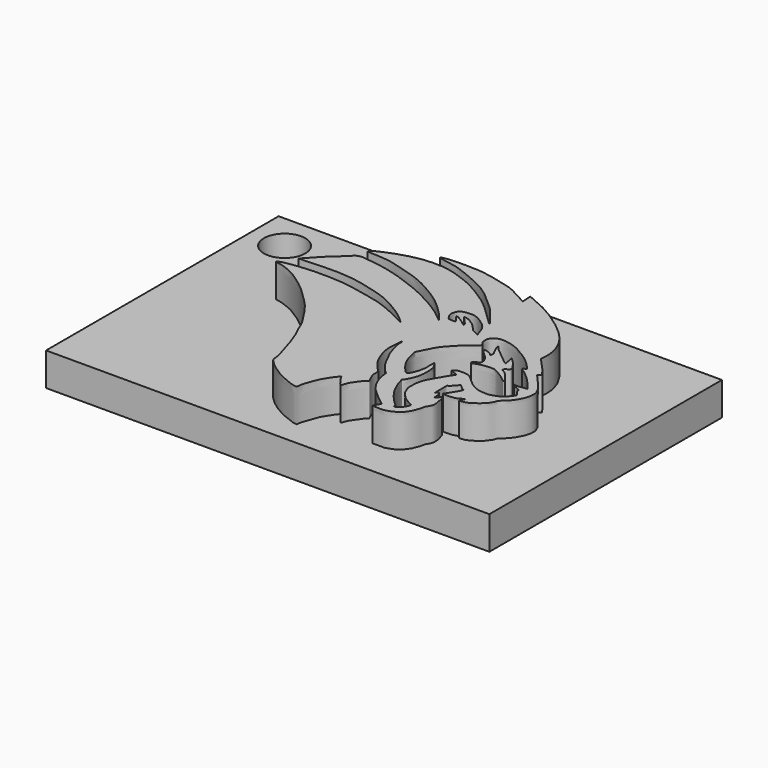
from build123d import *

# Parameters (mm, degrees)
F1_DEPTH = 25.4
F2_W     = 169.9344962835
F2_H     = 111.438959837
F3_DEPTH = 12.7
F4_R     = 7.9340721322
F5_DEPTH = 12.7


with BuildPart() as f1:
    # F0 (on Top) → F1 (new body)
    with BuildSketch(Plane.XY):
        with BuildLine():
            add(Edge.make_bspline(
                [(-14.8701705039, -19.9608001858), (-15.221690835, -19.2073334084), (-16.625382793, -16.9660551756), (-18.8145764823, -13.5974487599), (-21.7376055558, -9.4480503555), (-24.5386587115, -6.7651875872), (-29.2213836952, -2.0490323537), (-33.2090632506, 1.0266070698), (-37.3108516979, 3.8703194609), (-40.8750632464, 5.4725585398), (-43.1505063811, 6.3712258286), (-45.6984791671, 6.6961246185), (-46.2951241921, 7.0290269329), (-44.8273788111, 7.882301282), (-39.360546355, 8.6917755145), (-34.1503227711, 9.2199630692), (-26.1459287774, 9.1377803946), (-20.0552998643, 8.7078848215), (-11.5265680921, 6.7838277487), (-3.8234144736, 5.439385618), (7.2025946105, -0.1900501111), (7.7620278934, -0.5655499869), (4.9446039361, 2.0869717823), (1.3008896446, 4.7134534316), (-6.2511301784, 9.1315364238), (-13.4707319379, 10.9498852738), (-20.6605380633, 12.8767111483), (-30.7241335125, 13.5705283972), (-42.4874100153, 12.5018346524), (-41.7984071827, 12.9505929764), (-37.5569983073, 18.1037160515), (-31.7015431097, 22.7550582109), (-29.4633653878, 25.8033399973), (-24.708812529, 25.0026945191), (-20.5160586827, 24.5677127931), (-15.2447575815, 23.3952223693), (-11.1346154852, 22.1707374066), (-6.0005872173, 20.2473769611), (-1.6724236886, 18.5603562875), (2.331046156, 16.6096027421), (8.29978858, 13.3578117406), (12.9239596286, 10.140973274), (15.6933934459, 7.6938469217), (15.6850383581, 7.89041196), (13.883384297, 10.090120142), (12.2058740691, 12.0633831707), (8.2658950795, 15.7571136876), (5.1340905457, 18.2144922263), (0.5632813688, 21.0207749349), (-6.4295798331, 25.0167682013), (-16.519293927, 27.6010671806), (-19.6579640118, 28.5861202918), (-23.8244520748, 28.9321353102), (-27.5500194279, 29.1854619589), (-29.16994936, 29.0672202828), (-28.1023726327, 30.353145993), (-24.7800008778, 32.0217797709), (-18.8741048653, 34.1780204807), (-13.5989570646, 35.3844069692), (-9.0323236761, 35.7835224645), (-2.9568390979, 35.6441536417), (3.3871239944, 33.4430463754), (8.2582535453, 31.6254999822), (14.6988445903, 27.7308645526), (19.9782008784, 24.093188458), (24.8414343333, 19.1570210972), (29.0842273756, 15.1532805254), (29.0583545521, 15.3743411164), (27.8326579227, 17.2644078083), (25.9216038578, 19.4174660639), (23.0912459993, 23.2704910801), (19.4803048629, 26.0157171151), (16.9172953139, 28.7464960896), (12.009652843, 32.3100804683), (7.8786740384, 34.205264408), (-0.2201321112, 37.689521901), (-3.738465721, 38.5113119793), (-9.5098774215, 39.3772960778), (-9.2770451577, 39.8608323233), (-6.9503719579, 40.6697590859), (2.1658518543, 40.6240338322), (8.3670057819, 40.2357657644), (15.9816872911, 38.1517431998), (20.0146961816, 37.4251070757), (27.8026964381, 32.7643186249), (27.6739209409, 32.9274427311), (27.3919925021, 36.7329457257), (27.5484843103, 36.8192611002), (32.4487131354, 34.6740896565), (36.6415975911, 32.7362745493), (42.7969610095, 28.7852221639), (48.5775150448, 24.268635265), (52.9337999958, 19.280053861), (55.0956073548, 13.8730755246), (55.4842683059, 10.1023036419), (55.0875139263, 7.1366526371), (55.3311692316, 7.1202657281), (57.7038333216, 4.5151308529), (60.3403166523, 1.7873756635), (61.939783591, -0.7081872431), (61.9228089872, -0.8086404409), (60.574069747, -1.7619053144), (61.0873702539, -1.7516944394), (63.4024083186, -4.654014828), (66.17166014, -7.5165247573), (68.1323436188, -10.9753429081), (67.8403103062, -13.1464579427), (67.6210421965, -15.0307386106), (65.640256939, -18.8574840013), (63.7104902718, -20.7455148396), (61.9313019034, -22.131081262), (62.1416817304, -22.4638249746), (60.8967608126, -25.0173278873), (58.6701119256, -26.9078061444), (55.6505064167, -29.1445212539), (52.9064282632, -29.200166737), (52.8306873093, -28.9601536167), (54.2587664847, -26.6717106228), (53.8839650384, -27.2313234607), (51.986947732, -28.202550438), (50.6863481156, -28.8914707136), (46.3013264955, -28.9387192384), (46.5333158111, -28.5869206357), (50.3248376243, -22.7564692567), (49.2210127604, -22.7158735399), (48.185540697, -22.0953245327), (47.1820811341, -20.9209510008), (47.0179091111, -20.9423835074), (46.6610780555, -21.5222448894), (45.2715282704, -23.1642257164), (44.167485725, -23.8633478866), (44.0402199406, -24.056182696), (44.1077165563, -29.7391059746), (44.2424677108, -29.704882972), (44.9298643008, -28.6712101943), (44.9381784477, -28.8370782507), (45.5831789496, -29.401201917), (45.864978196, -30.2230405033), (45.8332800239, -32.2718499355), (46.0431048441, -32.2755521981), (47.4692449016, -30.6316210775), (47.5469474527, -30.6892542641), (48.1762281967, -31.282144751), (48.371150022, -32.9354354483), (49.2512481663, -36.4603778502), (47.3811785445, -38.5688666877), (47.4524172153, -39.4615142051), (46.5083937337, -42.4569406109), (44.8959673155, -45.3657836507), (41.914363728, -47.2577489049), (39.0930786202, -48.2934718337), (34.795474344, -47.9571483407), (34.6768461287, -47.8599376798), (36.1959801627, -45.3084678781), (36.1902562655, -45.2579861076), (33.7606289335, -43.4890994336), (31.005504084, -41.0736791631), (29.0903946087, -39.4485380637), (27.0544984579, -36.7124973539), (26.2052841843, -34.8407220549), (25.3516880158, -32.9031814643), (24.8613111568, -30.2531084511), (24.8021921451, -28.8153721599), (24.6122776651, -28.8230825397), (23.104162879, -27.4433091425), (21.7153959083, -25.6768723498), (20.4329502947, -23.8892225341), (18.6964093559, -20.1452708334), (17.2594231542, -17.5956807998), (16.6237447114, -14.5308822773), (15.7251002718, -12.5388593615), (15.9159556833, -9.7175450977), (15.5207961884, -9.7228985059), (15.3609709913, -13.0420997075), (15.0656157152, -16.1703142138), (16.0186872903, -20.1187864391), (17.4136983079, -23.5588760784), (18.9549102776, -25.9436355229), (21.9758647632, -29.3687856007), (22.3569011856, -29.4518910165), (22.2376625902, -31.1794785211), (22.4750841628, -33.0583982423), (24.0202604041, -35.8112373772), (23.9463212602, -36.028333464), (22.5757336735, -36.9887746178), (20.943115437, -39.6377331191), (19.7932835549, -40.972712028), (19.3189891957, -43.2705295118), (19.0892741552, -43.458963868), (18.4627295862, -43.0816932453), (17.8686520769, -42.1261702125), (17.0528733375, -41.1679156433), (16.109135116, -39.7611917977), (15.6583942757, -38.8552512589), (15.6104844294, -38.9871019848), (14.3312472417, -40.4613756955), (13.3504238678, -41.9874928854), (11.8584359055, -44.2493834769), (11.0665219392, -46.3231070406), (10.3429374422, -48.4545552842), (9.5481856978, -50.5759957274), (9.4060648235, -52.6403351753), (9.2664064233, -52.548184411), (7.3118521794, -52.2554939359), (6.1305638917, -51.7591076991), (4.0715548368, -50.9332182637), (2.6639768562, -50.3066956696), (0.3932070477, -49.2283306871), (-0.8310979, -48.3336778562), (-2.7127827276, -47.1310762319), (-4.0555159667, -46.1714522576), (-5.3632720538, -45.0356818132), (-6.4975041884, -43.8850295891), (-7.182897798, -43.1226518866), (-7.380134713, -41.7532388731), (-7.4756957962, -39.8994589754), (-8.5070257448, -36.9732060036), (-9.2147602073, -34.1386657639), (-10.8225901787, -29.4048978612), (-12.0411906467, -26.0805747104), (-14.3615500092, -21.5481532407), (-14.6179117826, -20.5015045177), (-14.8701705039, -19.9608001858)],
                knots=[0, 0, 0, 0, 0.0049590764, 0.0106061426, 0.016680571, 0.0221570205, 0.0291463365, 0.035406483, 0.041507596, 0.0468596575, 0.0512669827, 0.0555951815, 0.0572286385, 0.0601650163, 0.0665969859, 0.0731046834, 0.0807298933, 0.0876144071, 0.0954411961, 0.1038200224, 0.1131017527, 0.1140904599, 0.118810238, 0.1250375053, 0.1330476617, 0.1405539476, 0.1478284981, 0.1572094569, 0.1658855329, 0.1669309593, 0.1738224901, 0.1816783163, 0.1866466719, 0.1922969184, 0.1980883273, 0.2043697068, 0.2101110067, 0.2164930184, 0.2223771807, 0.2281425874, 0.2352554764, 0.2421856215, 0.2468671041, 0.2473346344, 0.2516558946, 0.2564592041, 0.2627017487, 0.2682262867, 0.2744074888, 0.282384837, 0.2911494078, 0.2961304728, 0.3016781712, 0.3071340679, 0.3098696002, 0.3125796856, 0.3179116131, 0.324879731, 0.3312527163, 0.3370665617, 0.3437997703, 0.3508469281, 0.3571476255, 0.3645737848, 0.3715184541, 0.3791939238, 0.3852229214, 0.385690448, 0.3895207526, 0.3944300134, 0.4003918346, 0.4061884017, 0.4115376563, 0.4181101703, 0.4242049613, 0.4321048907, 0.4379816572, 0.4440887567, 0.4451444794, 0.4490539196, 0.4573399172, 0.4645212824, 0.4718608605, 0.4782035884, 0.485915255, 0.4863827815, 0.4917402097, 0.4925264925, 0.4984560343, 0.5048101093, 0.5121024041, 0.5195938822, 0.5266301668, 0.5331279162, 0.538695168, 0.543034523, 0.5439975213, 0.5488290373, 0.5547449555, 0.5590731578, 0.5599045546, 0.5631786289, 0.5642240637, 0.5692763645, 0.5751173705, 0.5804194282, 0.5842950202, 0.5880583314, 0.5936498687, 0.5984342584, 0.602204778, 0.6035864923, 0.607914847, 0.6128095051, 0.6182308748, 0.6223969879, 0.6234527164, 0.6276280473, 0.6287400235, 0.6326366055, 0.636509555, 0.6418817611, 0.6430348398, 0.6500227568, 0.651870568, 0.6550343659, 0.658344166, 0.659153963, 0.6612392578, 0.6654028881, 0.6683692991, 0.6700051711, 0.676433051, 0.6769005775, 0.6798574986, 0.6804134934, 0.6827741764, 0.6856180495, 0.6893619372, 0.6901717169, 0.6941813883, 0.6948425707, 0.6971056628, 0.700695022, 0.7058660708, 0.7101646546, 0.7126665176, 0.7173844792, 0.7224741508, 0.7274362617, 0.7325236684, 0.7379167078, 0.7386158231, 0.7432876129, 0.7439487953, 0.7483990214, 0.7538993845, 0.7582783917, 0.7632614867, 0.7671915517, 0.7711550361, 0.775803219, 0.7788079417, 0.7796956946, 0.7834272361, 0.7876800285, 0.7917488674, 0.7972703082, 0.8020637783, 0.8067614762, 0.8110937967, 0.8153825704, 0.8161923588, 0.8208585152, 0.8260444454, 0.8314992394, 0.8366829416, 0.8416135651, 0.8472610284, 0.8487320422, 0.8520050943, 0.8561718649, 0.8608311889, 0.8618869239, 0.8652254355, 0.8701156049, 0.8739784356, 0.8779832805, 0.8791663401, 0.881313675, 0.8842410479, 0.8873494754, 0.89107548, 0.8935398956, 0.8940958815, 0.8977306082, 0.9016935172, 0.9061340889, 0.9102387251, 0.9142950107, 0.9186718845, 0.9222837622, 0.9229449498, 0.9266313029, 0.9300288983, 0.9339769443, 0.9375023646, 0.9417549496, 0.9452196622, 0.949250475, 0.9528113421, 0.9564191576, 0.9598913133, 0.9626013979, 0.9657002356, 0.9694549995, 0.974203598, 0.9789962015, 0.9850087791, 0.9904260981, 0.9964412577, 1, 1, 1, 1], degree=3))
        make_face()
        with BuildLine():
            add(Edge.make_bspline(
                [(29.4968672097, -24.9577090144), (29.2522813062, -24.9043141851), (28.4812583162, -24.3288345548), (27.5929491341, -23.2719328433), (26.5229917254, -21.9955450296), (25.493437854, -20.5251037399), (24.6801994651, -18.8995632069), (23.7965645353, -16.7549151809), (23.5446819954, -15.2740390303), (22.8719216364, -12.7119711385), (23.1418972942, -12.5584518565), (24.0154471471, -10.7766411032), (24.8407424624, -9.0693079132), (25.7289367901, -7.3485281619), (26.6559375418, -5.7613972679), (27.9062254963, -4.402126541), (29.3948903999, -2.6292634603), (31.343901089, -0.7824786076), (33.0107668247, 0.5689504112), (36.0390233406, 3.1686364904), (35.9834240148, 3.2841340245), (35.6347872021, 3.8315916102), (35.005968941, 4.300492855), (34.7946306934, 4.9794904566), (34.5639802183, 5.7982686669), (34.6727768135, 7.0835200419), (34.8494314161, 7.7637528325), (35.94184202, 8.8377452141), (36.7700559773, 9.3848304088), (38.0363565573, 9.6500972977), (39.3511875283, 9.7145928207), (40.869122491, 9.4131606486), (42.3186128653, 9.1230203463), (44.026639396, 8.5857606938), (45.8727467194, 7.68829074), (47.8396434221, 6.5647391811), (49.8921781905, 5.215646461), (51.5848538888, 4.0321336566), (52.9695426633, 2.8273251949), (53.9756652747, 1.9079844198), (54.8974443301, 0.9258478712), (56.0933963356, -0.5431734266), (56.0207767113, -0.5670851704), (54.1235992374, -1.2246906294), (56.2822414189, -2.2455961102), (57.6365652943, -3.4384410011), (59.3846260322, -4.8281482901), (61.5253326842, -7.1508611227), (62.8766661704, -8.6414132572), (64.2432189508, -10.4720364135), (64.1997307341, -10.526147049), (59.7430846208, -11.0959072724), (59.7174238209, -10.9952495415), (59.6902079837, -11.4932703081), (59.9344673636, -11.454688787), (60.6232913696, -11.7775056805), (61.9410395375, -12.3229908584), (62.6393846502, -12.5961227275), (62.6889607213, -12.6094395811), (62.6625293454, -13.4198997169), (62.9036332557, -13.6998131955), (63.4146030144, -14.6248848381), (64.2644012778, -15.4843576067), (64.2703472473, -15.7514541503), (63.9234444764, -16.361517992), (63.4297453755, -17.0077291171), (62.7483134067, -17.9428439939), (61.9461286613, -18.6920912439), (60.8047053901, -19.4764804344), (59.610563815, -19.9893153206), (58.3977560095, -20.3972567855), (57.1621739162, -20.7127926969), (54.2515411403, -20.5373729033), (52.545532541, -20.0953776823), (51.4815664159, -19.5692402803), (49.810596204, -18.671860239), (48.4987708398, -17.5074042444), (47.2886545958, -16.4657526062), (45.9680404199, -15.1378893551), (44.7528113291, -14.4934294299), (44.0590602712, -14.2394496595), (41.5424638767, -14.1212587014), (40.1505333119, -14.2608331208), (38.9793963625, -15.4409237635), (39.1237154987, -15.4063690401), (41.8773489728, -16.5324190222), (41.8239116772, -16.6685628078), (40.7814556828, -18.1805789408), (39.8307999292, -19.7584860445), (38.1065802723, -22.8115033724), (36.8276457119, -24.8247273526), (36.0353024844, -27.1936372084), (35.8496389089, -29.0603054241), (35.7335787494, -32.1031719848), (36.2453574344, -33.2884937889), (36.8904467346, -35.167947655), (38.2553679411, -36.6942464133), (39.4521075695, -37.8586499835), (41.1618511172, -39.1545600075), (42.6344482129, -39.8792255326), (43.5349553427, -40.2601234265), (43.6672085696, -40.3228808223), (43.3143919959, -41.291093515), (42.7961663324, -42.4471597398), (41.9537717412, -43.4601082839), (39.9286333798, -44.6437510012), (39.9618076609, -44.5526966368), (40.2143745036, -43.8364478953), (40.3769174243, -43.7835236104), (39.7876396563, -43.1654184035), (38.7768422844, -42.3758353972), (37.5647722531, -41.1135438714), (35.985791676, -39.4389294723), (34.8617251798, -37.7398674458), (33.7240328862, -36.1555212265), (32.5232966552, -33.6359437906), (31.7177003126, -31.7152639125), (31.0803960041, -29.2030854921), (31.027858707, -29.0871536111), (31.9380822088, -28.4634787891), (32.6092110474, -26.791776108), (33.3562917023, -25.1762993701), (33.6960741144, -23.6231477851), (33.9665612048, -21.6674261934), (33.8939165999, -19.4673360972), (33.7027397946, -17.7752237335), (33.3178878557, -16.5192743382), (31.8672968177, -14.4640934143), (31.9505985192, -14.7443602135), (31.8170442568, -16.2400374977), (31.9924971318, -18.777125191), (31.7811989512, -19.7408665822), (31.528565593, -21.2958227698), (31.1066790709, -22.4766680866), (30.6997434225, -23.6613789894), (29.9457354274, -24.859026972), (29.6448590614, -24.9900166803), (29.4968672097, -24.9577090144)],
                knots=[0, 0, 0, 0, 0.006708734, 0.0144130343, 0.0226490646, 0.0311626116, 0.039890883, 0.0493826184, 0.057895195, 0.0677654799, 0.0709231679, 0.0795607269, 0.0887905781, 0.097612174, 0.1062196534, 0.11485172, 0.1246327534, 0.1348342225, 0.1452057541, 0.1573642731, 0.1589999693, 0.1639254641, 0.1697072445, 0.1749195449, 0.1808782163, 0.1880129868, 0.193429241, 0.2011293672, 0.2076153379, 0.2147148113, 0.2220925584, 0.2299864519, 0.237772496, 0.2462695547, 0.2554227104, 0.2650908387, 0.2751205536, 0.2843744603, 0.2929782354, 0.3002602254, 0.3082835034, 0.3165615666, 0.317684609, 0.3249480775, 0.3327687674, 0.3418661817, 0.351408113, 0.3626123005, 0.3725114042, 0.3814704885, 0.3825935316, 0.3961282686, 0.397072702, 0.4010824118, 0.4036885486, 0.4091333639, 0.417180781, 0.4223604778, 0.4234835209, 0.4289134912, 0.4330069073, 0.4396236854, 0.4465657437, 0.4495595445, 0.4546913699, 0.4606197317, 0.4674303071, 0.4741699253, 0.4816466722, 0.488986991, 0.4960523262, 0.5033082496, 0.514206795, 0.5227193748, 0.5295815911, 0.5383182275, 0.5468204757, 0.5549256413, 0.5637399519, 0.5710041943, 0.5765496675, 0.5864616594, 0.5946376019, 0.6020108916, 0.6034230767, 0.6143949758, 0.6162049256, 0.6243221211, 0.6336315891, 0.6454446706, 0.6555491241, 0.6653333321, 0.67437203, 0.6852890022, 0.6926242463, 0.7014522327, 0.7105702363, 0.7188843537, 0.7282076754, 0.7366805764, 0.742645227, 0.7444812104, 0.7505381602, 0.7578489963, 0.7658296409, 0.775006834, 0.7758982315, 0.7814648168, 0.783617228, 0.7888689744, 0.7963361757, 0.8048163339, 0.8145443315, 0.8236276266, 0.8325853264, 0.8430582674, 0.8530497307, 0.8628253522, 0.8646080832, 0.8706988281, 0.8795016982, 0.8880478532, 0.8960344579, 0.905024029, 0.9145835946, 0.9226851084, 0.9307244732, 0.9400188431, 0.9415627396, 0.9492835742, 0.9596791693, 0.9661358264, 0.9739811762, 0.9811886388, 0.9884938738, 0.9959407392, 1, 1, 1, 1], degree=3))
        make_face(mode=Mode.SUBTRACT)
        with BuildLine():
            add(Edge.make_bspline(
                [(20.6397492439, 14.123653993), (20.9231291787, 14.107879862), (21.8316466788, 13.93482722), (23.1814379486, 13.2319928397), (24.2685977622, 12.5031395213), (25.2851042185, 11.8029468382), (26.4551056622, 10.4876070808), (27.0116800828, 9.9606050571), (27.651520023, 9.0647820094), (27.6538790026, 9.0845364936), (30.3610957538, 7.7412480397), (30.524767696, 7.7040205885), (30.4572964756, 8.0451735726), (30.1223764768, 9.0581679563), (29.5146238145, 10.7117994099), (28.9519533833, 12.0465400778), (27.7826519006, 13.3927760879), (26.8076966332, 14.1959491787), (25.5528714349, 15.1491849512), (24.249629435, 15.8970217765), (22.9819249355, 16.5507416428), (21.4841487521, 16.9479582393), (19.0832462787, 16.799759965), (17.8153748373, 16.5130973878), (16.8876470254, 15.9476291337), (16.3799579835, 15.2221343774), (16.0716009629, 14.4413838238), (15.8556372224, 12.9644797308), (16.2875433013, 11.8733345043), (16.6705653081, 11.1557862317), (17.4821370215, 10.366983682), (17.3319115827, 10.0971338051), (20.2859489837, 10.0363455976), (20.185530873, 10.1749470183), (19.9675570561, 10.5040692491), (19.4825241559, 11.3400304848), (18.935412513, 11.8704385213), (18.4480258577, 12.6144128586), (18.1808939016, 13.0607831433), (18.1662521839, 13.1213895313), (18.9230205816, 13.0032916053), (20.5270821027, 12.0237739131), (21.4184918676, 11.3544149547), (23.3070051117, 9.9365483519), (23.4059621734, 10.0067156562), (23.570445725, 10.4381450188), (22.713484547, 11.3464290964), (21.8490601971, 12.439939261), (21.0915870868, 13.162654499), (20.4832637271, 13.7262687032), (20.2820910891, 14.1154974665), (20.4994081257, 14.1314659759), (20.6397492439, 14.123653993)],
                knots=[0, 0, 0, 0, 0.0219174374, 0.0475683716, 0.0708173516, 0.0939041468, 0.1205139827, 0.1401868477, 0.1600837492, 0.1653534685, 0.2008124754, 0.2076571385, 0.217722134, 0.239007014, 0.2664663476, 0.291465973, 0.3183248648, 0.3415738438, 0.3670705028, 0.3923260235, 0.4164048852, 0.4420135516, 0.4736679694, 0.4972224458, 0.5179653105, 0.5367596874, 0.5555540687, 0.5803353932, 0.6021502725, 0.6215010109, 0.6421494073, 0.6502891489, 0.6839470051, 0.6878717971, 0.700359946, 0.7206658082, 0.7389231189, 0.7587499787, 0.772779121, 0.775554368, 0.7914380911, 0.8195318583, 0.8441701281, 0.8740926579, 0.8790278226, 0.8908831431, 0.9131954446, 0.9380422583, 0.959174794, 0.9779907894, 0.9891456053, 1, 1, 1, 1], degree=3))
        make_face(mode=Mode.SUBTRACT)
    extrude(amount=F1_DEPTH)


with BuildPart() as f1b:
    # F0 (on Top) → F1, piece 2 (new body)
    with BuildSketch(Plane.XY):
        with BuildLine():
            add(Edge.make_bspline(
                [(38.4243587725, 1.1815563076), (38.5444208528, 1.2963066813), (39.3898852999, 1.178648096), (40.237693022, 0.7831449991), (41.2099753906, 0.5100931346), (42.0509297876, -0.8607842728), (42.0577534479, 1.1404835539), (41.8456326025, 1.3541790338), (41.4392083091, 2.2659330897), (40.8158937108, 3.2740384466), (39.9587029792, 5.400934778), (40.3438916924, 5.559596747), (40.9557679363, 4.5685702947), (42.058222985, 3.5310359368), (43.9023139846, 2.1004669801), (45.3899206439, 1.0135238951), (49.2893968242, -2.554044408), (48.5479135699, -0.4179459769), (48.4310104839, 0.6853040701), (48.0367588725, 1.8763851572), (48.3293133891, 2.0403491265), (49.0636255934, 1.149349037), (50.067816964, 0.2972273841), (51.0134643651, -0.8712516698), (53.1529562448, -3.8841356631), (50.9330343922, -4.4175672132), (50.3822946155, -5.6227209917), (52.3408465011, -6.2703344725), (53.8960705123, -8.38330604), (55.5661312048, -10.1698195749), (55.4380832865, -11.1680266883), (54.6189284444, -10.4825853915), (53.6760464225, -9.7007174474), (52.5270377492, -8.8771483596), (51.4082367324, -8.1879749345), (50.0800058881, -7.3851648082), (48.76745003, -6.7450028476), (48.2700107452, -6.634105228), (47.3352057733, -6.5707134313), (45.9996521605, -6.6315669378), (44.1677165517, -6.8711792915), (42.4880173933, -7.2485387088), (39.9522354854, -8.3089250687), (40.72352612, -6.428408433), (42.3901546428, -6.3259765792), (42.74899106, -5.4903371237), (42.7064128818, -4.4189527249), (42.1474683351, -3.1361081469), (40.7240810395, -1.5240038795), (39.3475727947, -0.4781877099), (38.6148098913, 0.4209879463), (38.4228671185, 0.8189229514), (38.3510541927, 1.1114948203), (38.4243587725, 1.1815563076)],
                knots=[0, 0, 0, 0, 0.0161684258, 0.0337666663, 0.0518671601, 0.0682825224, 0.0882462774, 0.0989977666, 0.1150524213, 0.1359949613, 0.1610900016, 0.1679017618, 0.185324806, 0.2076732116, 0.2332411328, 0.2601235158, 0.2944900144, 0.3121937216, 0.3330035218, 0.3511834202, 0.3578609958, 0.3755288601, 0.3957384189, 0.4184251809, 0.448178711, 0.4702718078, 0.4866980007, 0.5090331223, 0.5383362424, 0.5654614676, 0.5782810189, 0.5933870872, 0.6135596773, 0.63414512, 0.6540813357, 0.6762195292, 0.6969079247, 0.7091780571, 0.7254500473, 0.7458210511, 0.7691241489, 0.7938248345, 0.8179471418, 0.8362177967, 0.8581434193, 0.8732682136, 0.8908120453, 0.9112952944, 0.9368598321, 0.9602188313, 0.9784205205, 0.9901282765, 1, 1, 1, 1], degree=3))
        make_face()
    extrude(amount=F1_DEPTH)


with BuildPart() as f3:
    # F2 (on Top) → F3 (new body)
    with BuildSketch(Plane.XY):
        with Locations((5.8495551348, -6.2461346388)):
            Rectangle(F2_W, F2_H)
    extrude(amount=F3_DEPTH)

    # F4 (on face) → F5 (cut, symmetric)
    with BuildSketch(Plane.XY.offset(12.7)):
        with Locations((-65.7331198454, 35.5930514634)):
            Circle(F4_R)
    extrude(amount=F5_DEPTH, both=True, mode=Mode.SUBTRACT)


solid = Compound([f1.part, f1b.part, f3.part])
